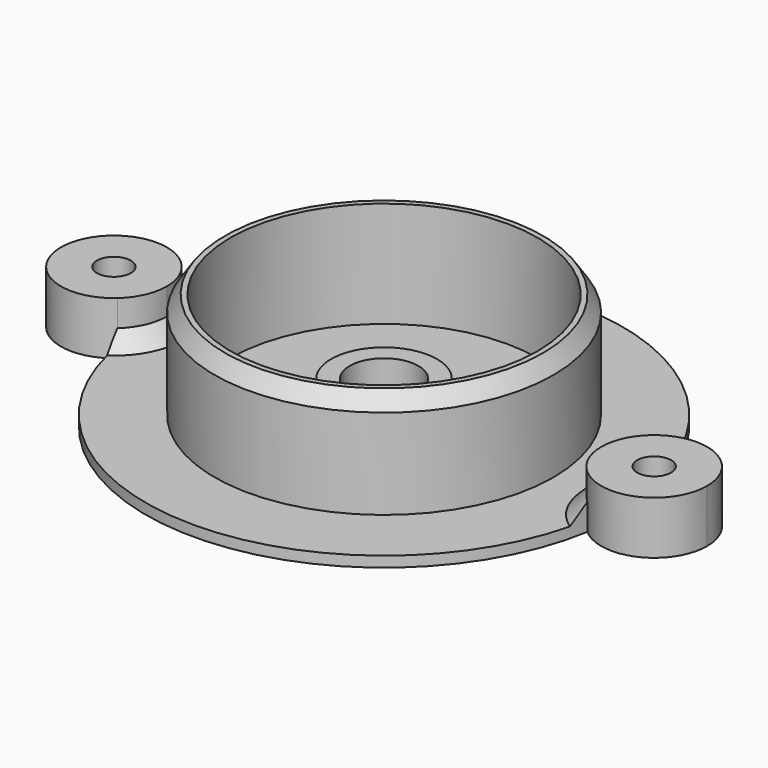
from build123d import *

# Parameters (mm, degrees)
F0_R         = 1.6
F1_DEPTH     = 5
F2_DEPTH     = 1
F3_R         = 16
F3_R_2       = 14.5
F4_DEPTH     = 10
F5_SIZE2     = 1.5
F5_SIZE      = 1
F8_T4_ANGLE  = 185.4300536725
F8_S5_R      = 22.5
F8_T6_DEPTH  = 9
F8_T10_ANGLE = 185.4300536725
F8_S11_R     = 22.5
F8_T12_DEPTH = 9
F9_R         = 5
F10_DEPTH    = 3
F11_R        = 3.25
F12_DEPTH    = 5


# Not quite as in the source:
# - a fillet or chamfer that OpenCascade refuses, or shapes differently, is made with other operations: its cross-section is extruded or revolved along the edge and cut away or added
# - a feature of the source that left no trace in its solid (it failed there, or was rolled back) is left out


with BuildPart() as f1:
    # F0 (on Top) → F1 (new body)
    with BuildSketch(Plane.XY):
        with BuildLine():
            ThreePointArc((-22.1862745098, -3.7442253372), (-22.5, 0), (-22.1862745098, 3.7442253372))
            ThreePointArc((-22.1862745098, 3.7442253372), (-30.5, 0), (-22.1862745098, -3.7442253372))
        make_face()
        with Locations((-25.5, 0)):
            Circle(F0_R, mode=Mode.SUBTRACT)
        with BuildLine():
            ThreePointArc((-20.5, 0), (-20.9410183456, 2.0532136456), (-22.1862745098, 3.7442253372))
            ThreePointArc((-22.1862745098, 3.7442253372), (-22.5, 0), (-22.1862745098, -3.7442253372))
            ThreePointArc((-22.1862745098, -3.7442253372), (-20.9410183456, -2.0532136456), (-20.5, 0))
        make_face()
    extrude(amount=F1_DEPTH)



with BuildPart() as f1b:
    # F0 (on Top) → F1, piece 2 (new body)
    with BuildSketch(Plane.XY):
        with BuildLine():
            ThreePointArc((22.1862745098, 3.7442253372), (22.4214314493, 1.8786728733), (22.5, 0))
            ThreePointArc((22.5, 0), (22.4214314493, -1.8786728733), (22.1862745098, -3.7442253372))
            ThreePointArc((22.1862745098, -3.7442253372), (27.5532136456, -4.5589816544), (30.5, 0))
            ThreePointArc((30.5, 0), (27.5532136456, 4.5589816544), (22.1862745098, 3.7442253372))
        make_face()
        with Locations((25.5, 0)):
            Circle(F0_R, mode=Mode.SUBTRACT)
        with BuildLine():
            ThreePointArc((22.1862745098, -3.7442253372), (22.4214314493, -1.8786728733), (22.5, 0))
            ThreePointArc((22.5, 0), (22.4214314493, 1.8786728733), (22.1862745098, 3.7442253372))
            ThreePointArc((22.1862745098, 3.7442253372), (20.5, 0), (22.1862745098, -3.7442253372))
        make_face()
    extrude(amount=F1_DEPTH)


with BuildPart() as f1_1:
    add(f1.part)

    add(f1b.part)  # F2 merges F1b
    # F0 (on Top) → F2 (join)
    with BuildSketch(Plane.XY):
        with BuildLine():
            ThreePointArc((22.1862745098, -3.7442253372), (20.5, 0), (22.1862745098, 3.7442253372))
            ThreePointArc((22.1862745098, 3.7442253372), (0, 22.5), (-22.1862745098, 3.7442253372))
            ThreePointArc((-22.1862745098, 3.7442253372), (-20.9410183456, 2.0532136456), (-20.5, 0))
            ThreePointArc((-20.5, 0), (-20.9410183456, -2.0532136456), (-22.1862745098, -3.7442253372))
            ThreePointArc((-22.1862745098, -3.7442253372), (0, -22.5), (22.1862745098, -3.7442253372))
        make_face()
    extrude(amount=F2_DEPTH)

    # F3 (on face) → F4 (join)
    with BuildSketch(Plane.XY.offset(1)):
        Circle(F3_R)
        Circle(F3_R_2, mode=Mode.SUBTRACT)
    extrude(amount=F4_DEPTH)

    # F5
    f5_edges = [f1_1.edges().sort_by_distance(p)[0] for p in [
        (-16, 0, 11),
    ]]
    f5_side = f1_1.faces().sort_by_distance((-15.547452, 0, 11))[0]
    chamfer(f5_edges, length=F5_SIZE, length2=F5_SIZE2, reference=f5_side)

    # F8: chamfer of 1.5 on 2 edges, made by hand


with BuildPart() as f8_tool2:
    # F8_s3 → F8_t4 (revolve)
    with BuildSketch(Plane(origin=(25.4427839223, 1.2065389767, 0), x_dir=(0, 0, 1), z_dir=(0.9988774861, 0.0473684257, 0))):
        Polygon((1, 7.7078948555), (2.5, 6.2078948555), (1, 6.2078948555), align=None)
    revolve(axis=Axis((25.5, 0, 1), (0, 0, -1)), revolution_arc=F8_T4_ANGLE)

    # F8_s5 → F8_t6 (intersect, symmetric)
    with BuildSketch(Plane.XY.offset(1.8)):
        Circle(F8_S5_R)
    extrude(amount=F8_T6_DEPTH, both=True, mode=Mode.INTERSECT)


with BuildPart() as f1_2:
    add(f1_1.part)

    # F8_t1: union F8_tool2
    add(f8_tool2.part)


with BuildPart() as f8_tool8:
    # F8_s9 → F8_t10 (revolve)
    with BuildSketch(Plane(origin=(-25.4427839223, 1.2065389767, 0), x_dir=(0, 0, 1), z_dir=(-0.9988774861, 0.0473684257, 0))):
        Polygon((1, -7.7078948555), (2.5, -6.2078948555), (1, -6.2078948555), align=None)
    revolve(axis=Axis((-25.5, 0, 1), (0, 0, 1)), revolution_arc=F8_T10_ANGLE)

    # F8_s11 → F8_t12 (intersect, symmetric)
    with BuildSketch(Plane.XY.offset(1.7)):
        Circle(F8_S11_R)
    extrude(amount=F8_T12_DEPTH, both=True, mode=Mode.INTERSECT)


with BuildPart() as f1_3:
    add(f1_2.part)

    # F8_t7: union F8_tool8
    add(f8_tool8.part)

    # F9 (on face) → F10 (join)
    with BuildSketch(Plane.XY.offset(1)):
        Circle(F9_R)
    extrude(amount=F10_DEPTH)

    # F11 (on face) → F12 (cut)
    with BuildSketch(Plane.XY.offset(4)):
        Circle(F11_R)
    extrude(amount=-F12_DEPTH, mode=Mode.SUBTRACT)


solid = f1_3.part
